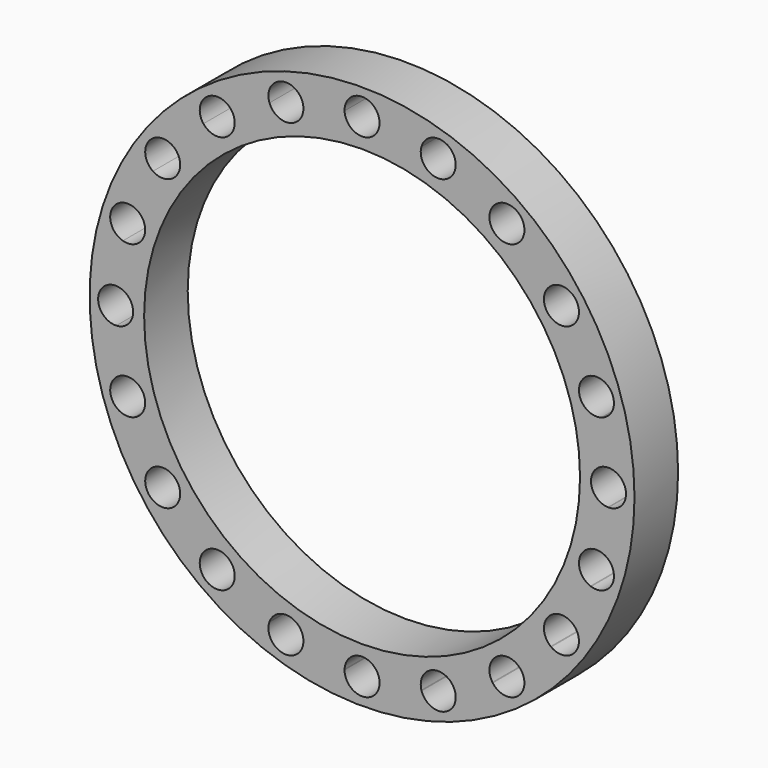
from build123d import *

# Parameters (mm, degrees)
F0_R            = 127
F1_DEPTH        = 25.4
F2_R            = 101.6
F3_DEPTH        = 25.401
F5_DEPTH        = 19.05
F5_COPIES_COUNT = 20


# Not quite as in the source:
# - a pattern or mirror of a feature is missing from the dataset's text; its kind, count and spacing are read off the source's solid


with BuildPart() as f1:
    # F0 (on Front) → F1 (new body)
    with BuildSketch(Plane.XZ):
        Circle(F0_R)
    extrude(amount=F1_DEPTH)

    # F2 (on face) → F3 (cut, through all)
    with BuildSketch(Plane.XZ.offset(25.4)):
        Circle(F2_R)
    extrude(amount=-F3_DEPTH, mode=Mode.SUBTRACT)

    # F4 (on face) → F5 (cut)
    with BuildSketch(Plane.XZ.offset(25.4)):
        with BuildLine():
            ThreePointArc((-8.1511862482, 114.5919902466), (0, 106.7252035251), (8.1511862482, 114.5919902466))
            ThreePointArc((8.1511862482, 114.5919902466), (0, 114.8815305693), (-8.1511862482, 114.5919902466))
        make_face()
        with BuildLine():
            ThreePointArc((-8.1511862482, 114.5919902466), (0, 114.8815305693), (8.1511862482, 114.5919902466))
            ThreePointArc((8.1511862482, 114.5919902466), (8.1550417439, 114.736737591), (8.1563270441, 114.8815305693))
            ThreePointArc((8.1563270441, 114.8815305693), (-0.1447929783, 123.0365723132), (-8.1511862482, 114.5919902466))
        make_face()
    f5 = extrude(amount=-F5_DEPTH, mode=Mode.SUBTRACT)

    # F5_copies: F5 ×20 about axis
    f5_copies_axis = Axis((0, 0, 0), (0, 1, 0))
    for i in range(1, F5_COPIES_COUNT):
        add(f5.rotate(f5_copies_axis, i * 360 / F5_COPIES_COUNT), mode=Mode.SUBTRACT)


solid = f1.part
